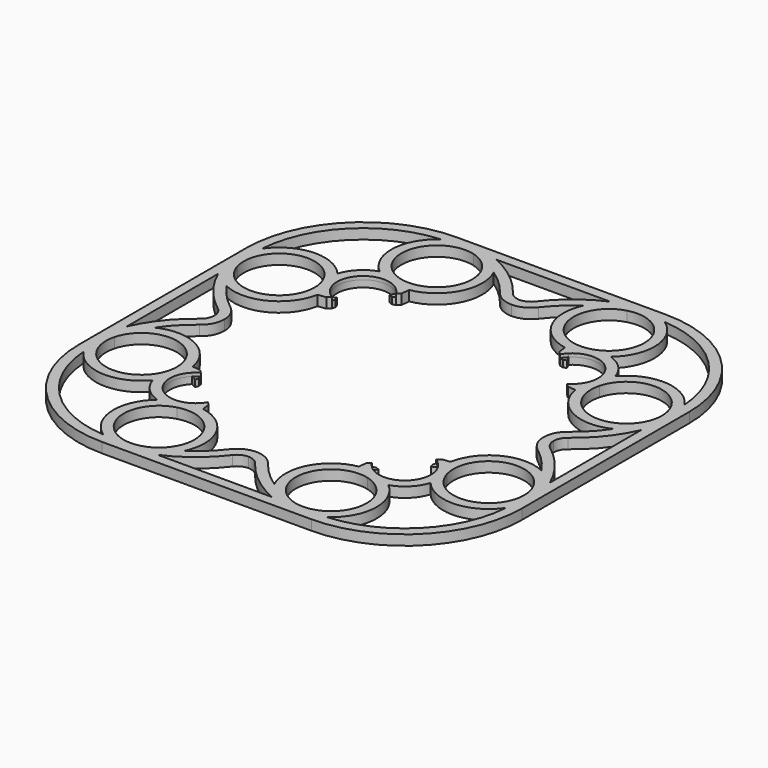
from build123d import *
from build123d import SkipClean  # not in build123d's __all__

# Parameters (mm, degrees)
F2_DEPTH = 1.5
F3_R     = 3.85
F4_DEPTH = 0.5


with BuildPart() as f2:
    # F1 (on Top) → F2 (new body)
    with BuildSketch(Plane.XY):
        with BuildLine():
            Line((0, 32.85), (-15.5, 32.85))
            ThreePointArc((-15.5, 32.85), (-27.7683026536, 27.7683026536), (-32.85, 15.5))
            Line((-32.85, 15.5), (-32.85, 0))
            Line((-32.85, 0), (-32.85, -15.5))
            ThreePointArc((-32.85, -15.5), (-27.7683026536, -27.7683026536), (-15.5, -32.85))
            Line((-15.5, -32.85), (0, -32.85))
            Line((0, -32.85), (15.5, -32.85))
            ThreePointArc((15.5, -32.85), (27.7683026536, -27.7683026536), (32.85, -15.5))
            Line((32.85, -15.5), (32.85, 0))
            Line((32.85, 0), (32.85, 15.5))
            ThreePointArc((32.85, 15.5), (27.7683026536, 27.7683026536), (15.5, 32.85))
            Line((15.5, 32.85), (0, 32.85))
        make_face()
        with BuildLine():
            ThreePointArc((-20.5960975648, -17.1285851559), (-19.2830212793, -19.2830212793), (-17.1285851559, -20.5960975648))
            ThreePointArc((-17.1285851559, -20.5960975648), (-19.4970773189, -26.0956914855), (-16.5611043163, -31.3144414264))
            ThreePointArc((-16.5611043163, -31.3144414264), (-26.7076424818, -26.7076424818), (-31.3144414264, -16.5611043163))
            ThreePointArc((-31.3144414264, -16.5611043163), (-26.0956914855, -19.4970773189), (-20.5960975648, -17.1285851559))
        make_face(mode=Mode.SUBTRACT)
        with BuildLine():
            ThreePointArc((-14.1153181087, -20.6677031706), (-9.5605206196, -21.5737087221), (-7.5065181219, -25.7388137587))
            ThreePointArc((-7.5065181219, -25.7388137587), (-8.5914130854, -28.934811261), (-11.3977181351, -30.8099243467))
            ThreePointArc((-11.3977181351, -30.8099243467), (-17.8276287099, -27.0976137455), (-14.1153181087, -20.6677031706))
        make_face(mode=Mode.SUBTRACT)
        with BuildLine():
            Line((0, -31.35), (-8.4430884942, -31.35))
            ThreePointArc((-8.4430884942, -31.35), (-4.7131487758, -29.0891994123), (-1.6649039264, -25.9696044163))
            ThreePointArc((-1.6649039264, -25.9696044163), (-0.9297120163, -25.3600434151), (0, -25.1416233484))
            ThreePointArc((0, -25.1416233484), (0.9297120163, -25.3600434151), (1.6649039264, -25.9696044163))
            ThreePointArc((1.6649039264, -25.9696044163), (4.7131487758, -29.0891994123), (8.4430884942, -31.35))
            Line((8.4430884942, -31.35), (0, -31.35))
        make_face(mode=Mode.SUBTRACT)
        with BuildLine():
            ThreePointArc((-30.8099243467, -11.3977181351), (-25.0535512495, -7.5514325997), (-20.4888137587, -12.7565181219))
            ThreePointArc((-20.4888137587, -12.7565181219), (-20.5337282365, -13.4417806311), (-20.6677031706, -14.1153181087))
            ThreePointArc((-20.6677031706, -14.1153181087), (-27.0976137455, -17.8276287099), (-30.8099243467, -11.3977181351))
        make_face(mode=Mode.SUBTRACT)
        with BuildLine():
            ThreePointArc((14.1153181087, -20.6677031706), (16.9216231584, -22.5428162564), (18.0065181219, -25.7388137587))
            ThreePointArc((18.0065181219, -25.7388137587), (15.9525156242, -29.9039187952), (11.3977181351, -30.8099243467))
            ThreePointArc((11.3977181351, -30.8099243467), (7.6854075339, -24.3800137719), (14.1153181087, -20.6677031706))
        make_face(mode=Mode.SUBTRACT)
        with BuildLine():
            ThreePointArc((17.1285851559, -20.5960975648), (19.2830212793, -19.2830212793), (20.5960975648, -17.1285851559))
            ThreePointArc((20.5960975648, -17.1285851559), (26.0956914855, -19.4970773189), (31.3144414264, -16.5611043163))
            ThreePointArc((31.3144414264, -16.5611043163), (26.7076424818, -26.7076424818), (16.5611043163, -31.3144414264))
            ThreePointArc((16.5611043163, -31.3144414264), (19.4970773189, -26.0956914855), (17.1285851559, -20.5960975648))
        make_face(mode=Mode.SUBTRACT)
        with BuildLine():
            ThreePointArc((30.8099243467, -11.3977181351), (30.9438992809, -12.0712556128), (30.9888137587, -12.7565181219))
            ThreePointArc((30.9888137587, -12.7565181219), (26.4240762678, -17.9616036441), (20.6677031706, -14.1153181087))
            ThreePointArc((20.6677031706, -14.1153181087), (24.3800137719, -7.6854075339), (30.8099243467, -11.3977181351))
        make_face(mode=Mode.SUBTRACT)
        with BuildLine():
            Line((31.35, 0), (31.35, -8.4430884942))
            ThreePointArc((31.35, -8.4430884942), (29.0891994123, -4.7131487758), (25.9696044163, -1.6649039264))
            ThreePointArc((25.9696044163, -1.6649039264), (25.3600434151, -0.9297120163), (25.1416233484, 0))
            ThreePointArc((25.1416233484, 0), (25.3600434151, 0.9297120163), (25.9696044163, 1.6649039264))
            ThreePointArc((25.9696044163, 1.6649039264), (29.0891994123, 4.7131487758), (31.35, 8.4430884942))
            Line((31.35, 8.4430884942), (31.35, 0))
        make_face(mode=Mode.SUBTRACT)
        with BuildLine():
            Line((-31.35, 0), (-31.35, 8.4430884942))
            ThreePointArc((-31.35, 8.4430884942), (-29.0891994123, 4.7131487758), (-25.9696044163, 1.6649039264))
            ThreePointArc((-25.9696044163, 1.6649039264), (-25.3600434151, 0.9297120163), (-25.1416233484, 0))
            ThreePointArc((-25.1416233484, 0), (-25.3600434151, -0.9297120163), (-25.9696044163, -1.6649039264))
            ThreePointArc((-25.9696044163, -1.6649039264), (-29.0891994123, -4.7131487758), (-31.35, -8.4430884942))
            Line((-31.35, -8.4430884942), (-31.35, 0))
        make_face(mode=Mode.SUBTRACT)
        with BuildLine():
            ThreePointArc((-30.8099243467, 11.3977181351), (-27.0976137455, 17.8276287099), (-20.6677031706, 14.1153181087))
            ThreePointArc((-20.6677031706, 14.1153181087), (-20.5337282365, 13.4417806311), (-20.4888137587, 12.7565181219))
            ThreePointArc((-20.4888137587, 12.7565181219), (-25.0535512495, 7.5514325997), (-30.8099243467, 11.3977181351))
        make_face(mode=Mode.SUBTRACT)
        with BuildLine():
            ThreePointArc((-16.5611043163, 31.3144414264), (-19.4970773189, 26.0956914855), (-17.1285851559, 20.5960975648))
            ThreePointArc((-17.1285851559, 20.5960975648), (-19.2830212793, 19.2830212793), (-20.5960975648, 17.1285851559))
            ThreePointArc((-20.5960975648, 17.1285851559), (-26.0956914855, 19.4970773189), (-31.3144414264, 16.5611043163))
            ThreePointArc((-31.3144414264, 16.5611043163), (-26.7076424818, 26.7076424818), (-16.5611043163, 31.3144414264))
        make_face(mode=Mode.SUBTRACT)
        with BuildLine():
            ThreePointArc((-7.5065181219, 25.7388137587), (-9.5605206196, 21.5737087221), (-14.1153181087, 20.6677031706))
            ThreePointArc((-14.1153181087, 20.6677031706), (-17.8276287099, 27.0976137455), (-11.3977181351, 30.8099243467))
            ThreePointArc((-11.3977181351, 30.8099243467), (-8.5914130854, 28.934811261), (-7.5065181219, 25.7388137587))
        make_face(mode=Mode.SUBTRACT)
        with BuildLine():
            ThreePointArc((-6.6738359928, 28.6651558638), (-4.6174749504, 27.023590957), (-2.8610217426, 25.0644512968))
            ThreePointArc((-2.8610217426, 25.0644512968), (-1.5976455162, 24.0169630603), (0, 23.6416233484))
            ThreePointArc((0, 23.6416233484), (1.5976455162, 24.0169630603), (2.8610217426, 25.0644512968))
            ThreePointArc((2.8610217426, 25.0644512968), (4.6174749504, 27.023590957), (6.6738359928, 28.6651558638))
            ThreePointArc((6.6738359928, 28.6651558638), (6.7405837582, 22.6775993376), (11.5415551004, 19.0990573734))
            Line((11.5415551004, 19.0990573734), (11.6904748073, 17.8953116303))
            Line((11.6904748073, 17.8953116303), (12.1639675827, 17.4218188549))
            Line((12.1639675827, 17.4218188549), (12.6779191196, 17.3015221953))
            Line((12.6779191196, 17.3015221953), (13.1549797952, 17.4737945199))
            Line((13.1549797952, 17.4737945199), (12.7776388924, 18.2223611076))
            ThreePointArc((12.7776388924, 18.2223611076), (18.2223611076, 18.2223611076), (18.2223611076, 12.7776388924))
            Line((18.2223611076, 12.7776388924), (17.4737945199, 13.1549797952))
            Line((17.4737945199, 13.1549797952), (17.3015221953, 12.6779191196))
            Line((17.3015221953, 12.6779191196), (17.4218188549, 12.1639675827))
            Line((17.4218188549, 12.1639675827), (17.8953116303, 11.6904748073))
            Line((17.8953116303, 11.6904748073), (19.0990573734, 11.5415551004))
            ThreePointArc((19.0990573734, 11.5415551004), (22.6775993376, 6.7405837582), (28.6651558638, 6.6738359928))
            ThreePointArc((28.6651558638, 6.6738359928), (27.023590957, 4.6174749504), (25.0644512968, 2.8610217426))
            ThreePointArc((25.0644512968, 2.8610217426), (24.0169630603, 1.5976455162), (23.6416233484, 0))
            ThreePointArc((23.6416233484, 0), (24.0169630603, -1.5976455162), (25.0644512968, -2.8610217426))
            ThreePointArc((25.0644512968, -2.8610217426), (27.023590957, -4.6174749504), (28.6651558638, -6.6738359928))
            ThreePointArc((28.6651558638, -6.6738359928), (22.6775993376, -6.7405837582), (19.0990573734, -11.5415551004))
            Line((19.0990573734, -11.5415551004), (17.8953116303, -11.6904748073))
            Line((17.8953116303, -11.6904748073), (17.4218188549, -12.1639675827))
            Line((17.4218188549, -12.1639675827), (17.3015221953, -12.6779191196))
            Line((17.3015221953, -12.6779191196), (17.4737945199, -13.1549797952))
            Line((17.4737945199, -13.1549797952), (18.2223611076, -12.7776388924))
            ThreePointArc((18.2223611076, -12.7776388924), (18.2223611076, -18.2223611076), (12.7776388924, -18.2223611076))
            Line((12.7776388924, -18.2223611076), (13.1549797952, -17.4737945199))
            Line((13.1549797952, -17.4737945199), (12.6779191196, -17.3015221953))
            Line((12.6779191196, -17.3015221953), (12.1639675827, -17.4218188549))
            Line((12.1639675827, -17.4218188549), (11.6904748073, -17.8953116303))
            Line((11.6904748073, -17.8953116303), (11.5415551004, -19.0990573734))
            ThreePointArc((11.5415551004, -19.0990573734), (6.7405837582, -22.6775993376), (6.6738359928, -28.6651558638))
            ThreePointArc((6.6738359928, -28.6651558638), (4.6174749504, -27.023590957), (2.8610217426, -25.0644512968))
            ThreePointArc((2.8610217426, -25.0644512968), (1.5976455162, -24.0169630603), (0, -23.6416233484))
            ThreePointArc((0, -23.6416233484), (-1.5976455162, -24.0169630603), (-2.8610217426, -25.0644512968))
            ThreePointArc((-2.8610217426, -25.0644512968), (-4.6174749504, -27.023590957), (-6.6738359928, -28.6651558638))
            ThreePointArc((-6.6738359928, -28.6651558638), (-6.7405837582, -22.6775993376), (-11.5415551004, -19.0990573734))
            Line((-11.5415551004, -19.0990573734), (-11.6904748073, -17.8953116303))
            Line((-11.6904748073, -17.8953116303), (-12.1639675827, -17.4218188549))
            Line((-12.1639675827, -17.4218188549), (-12.6779191196, -17.3015221953))
            Line((-12.6779191196, -17.3015221953), (-13.1549797952, -17.4737945199))
            Line((-13.1549797952, -17.4737945199), (-12.7776388924, -18.2223611076))
            ThreePointArc((-12.7776388924, -18.2223611076), (-18.2223611076, -18.2223611076), (-18.2223611076, -12.7776388924))
            Line((-18.2223611076, -12.7776388924), (-17.4737945199, -13.1549797952))
            Line((-17.4737945199, -13.1549797952), (-17.3015221953, -12.6779191196))
            Line((-17.3015221953, -12.6779191196), (-17.4218188549, -12.1639675827))
            Line((-17.4218188549, -12.1639675827), (-17.8953116303, -11.6904748073))
            Line((-17.8953116303, -11.6904748073), (-19.0990573734, -11.5415551004))
            ThreePointArc((-19.0990573734, -11.5415551004), (-22.6775993376, -6.7405837582), (-28.6651558638, -6.6738359928))
            ThreePointArc((-28.6651558638, -6.6738359928), (-27.023590957, -4.6174749504), (-25.0644512968, -2.8610217426))
            ThreePointArc((-25.0644512968, -2.8610217426), (-24.0169630603, -1.5976455162), (-23.6416233484, 0))
            ThreePointArc((-23.6416233484, 0), (-24.0169630603, 1.5976455162), (-25.0644512968, 2.8610217426))
            ThreePointArc((-25.0644512968, 2.8610217426), (-27.023590957, 4.6174749504), (-28.6651558638, 6.6738359928))
            ThreePointArc((-28.6651558638, 6.6738359928), (-22.6775993376, 6.7405837582), (-19.0990573734, 11.5415551004))
            Line((-19.0990573734, 11.5415551004), (-17.8953116303, 11.6904748073))
            Line((-17.8953116303, 11.6904748073), (-17.4218188549, 12.1639675827))
            Line((-17.4218188549, 12.1639675827), (-17.3015221953, 12.6779191196))
            Line((-17.3015221953, 12.6779191196), (-17.4737945199, 13.1549797952))
            Line((-17.4737945199, 13.1549797952), (-18.2223611076, 12.7776388924))
            ThreePointArc((-18.2223611076, 12.7776388924), (-18.2223611076, 18.2223611076), (-12.7776388924, 18.2223611076))
            Line((-12.7776388924, 18.2223611076), (-13.1549797952, 17.4737945199))
            Line((-13.1549797952, 17.4737945199), (-12.6779191196, 17.3015221953))
            Line((-12.6779191196, 17.3015221953), (-12.1639675827, 17.4218188549))
            Line((-12.1639675827, 17.4218188549), (-11.6904748073, 17.8953116303))
            Line((-11.6904748073, 17.8953116303), (-11.5415551004, 19.0990573734))
            ThreePointArc((-11.5415551004, 19.0990573734), (-6.7405837582, 22.6775993376), (-6.6738359928, 28.6651558638))
        make_face(mode=Mode.SUBTRACT)
        with BuildLine():
            ThreePointArc((20.6677031706, 14.1153181087), (26.4240762678, 17.9616036441), (30.9888137587, 12.7565181219))
            ThreePointArc((30.9888137587, 12.7565181219), (30.9438992809, 12.0712556128), (30.8099243467, 11.3977181351))
            ThreePointArc((30.8099243467, 11.3977181351), (24.3800137719, 7.6854075339), (20.6677031706, 14.1153181087))
        make_face(mode=Mode.SUBTRACT)
        with BuildLine():
            ThreePointArc((-1.6649039264, 25.9696044163), (-4.7131487758, 29.0891994123), (-8.4430884942, 31.35))
            Line((-8.4430884942, 31.35), (0, 31.35))
            Line((0, 31.35), (8.4430884942, 31.35))
            ThreePointArc((8.4430884942, 31.35), (4.7131487758, 29.0891994123), (1.6649039264, 25.9696044163))
            ThreePointArc((1.6649039264, 25.9696044163), (0.9297120163, 25.3600434151), (0, 25.1416233484))
            ThreePointArc((0, 25.1416233484), (-0.9297120163, 25.3600434151), (-1.6649039264, 25.9696044163))
        make_face(mode=Mode.SUBTRACT)
        with BuildLine():
            ThreePointArc((11.3977181351, 30.8099243467), (15.9525156242, 29.9039187952), (18.0065181219, 25.7388137587))
            ThreePointArc((18.0065181219, 25.7388137587), (16.9216231584, 22.5428162564), (14.1153181087, 20.6677031706))
            ThreePointArc((14.1153181087, 20.6677031706), (7.6854075339, 24.3800137719), (11.3977181351, 30.8099243467))
        make_face(mode=Mode.SUBTRACT)
        with BuildLine():
            ThreePointArc((20.5960975648, 17.1285851559), (19.2830212793, 19.2830212793), (17.1285851559, 20.5960975648))
            ThreePointArc((17.1285851559, 20.5960975648), (19.4970773189, 26.0956914855), (16.5611043163, 31.3144414264))
            ThreePointArc((16.5611043163, 31.3144414264), (26.7076424818, 26.7076424818), (31.3144414264, 16.5611043163))
            ThreePointArc((31.3144414264, 16.5611043163), (26.0956914855, 19.4970773189), (20.5960975648, 17.1285851559))
        make_face(mode=Mode.SUBTRACT)
    extrude(amount=F2_DEPTH)

    # F3 (on face) → F4 (cut)
    with BuildSketch(Plane.XY.offset(1.5)):
        with Locations((-15.5, 15.5)):
            Circle(F3_R)
        with Locations((15.5, 15.5)):
            Circle(F3_R)
        with Locations((15.5, -15.5)):
            Circle(F3_R)
        with Locations((-15.5, -15.5)):
            Circle(F3_R)
    with SkipClean():  # cleaning this boolean's faces spoils the solid; the shape is the same uncleaned
        extrude(amount=-F4_DEPTH, mode=Mode.SUBTRACT)


solid = f2.part
